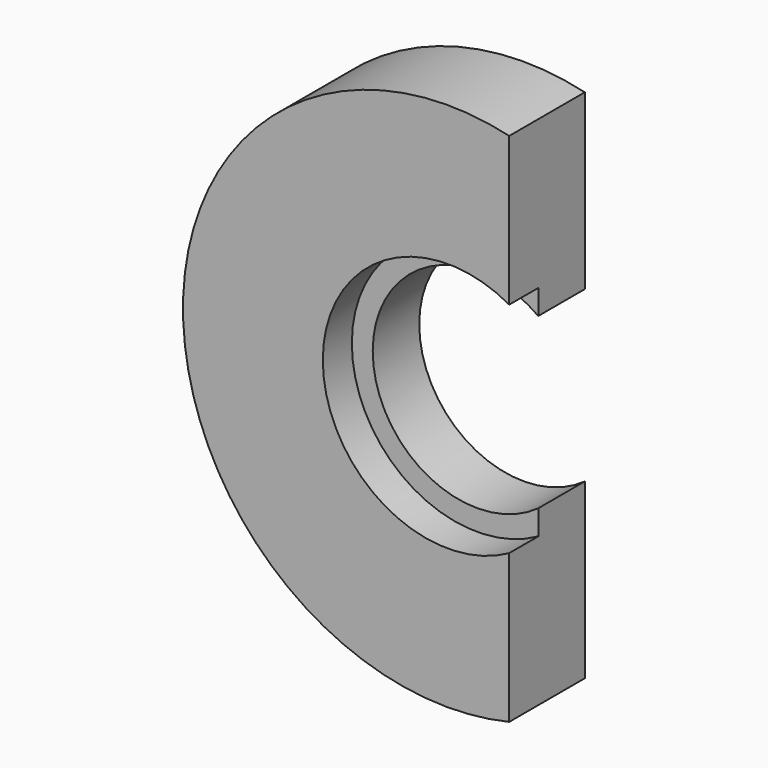
from build123d import *

# Parameters (mm, degrees)
F6_DEPTH = 9.501


# Not quite as in the source:
# - a feature of the source that left no trace in its solid (it failed there, or was rolled back) is left out
# - the program builds the solid bodies; features that only make, move or delete a surface that nothing else refers to are left out


with BuildPart() as f4:
    # F0 (on Top) → F4 (revolve)
    with BuildSketch(Plane.XY):
        Polygon((34.4624469289, 70.1398981537), (36.5624469289, 70.1398981537), (36.5624469289, 75.9898981537), (20.4008240253, 75.9898981537), (20.4008240253, 66.4898981537), (28.4008240253, 66.4898981537), (34.4624469289, 66.4898981537), align=None)
    revolve(axis=Axis((47.0624469289, 47.4898981537, 0), (0, -1, 0)))

    # F5 (on face) → F6 (cut, through all)
    with BuildSketch(Plane(origin=(0, 75.9898981537, 0), x_dir=(-1, 0, 0), z_dir=(0, 1, 0))):
        with BuildLine():
            Line((-53.2110722647, 8.511427993), (-53.2110722647, 25.9429478343))
            ThreePointArc((-53.2110722647, 25.9429478343), (-73.7240698325, 0), (-53.2110722647, -25.9429478343))
            Line((-53.2110722647, -25.9429478343), (-53.2110722647, -8.511427993))
            ThreePointArc((-53.2110722647, -8.511427993), (-57.5624469289, 0), (-53.2110722647, 8.511427993))
        make_face()
    extrude(amount=-F6_DEPTH, mode=Mode.SUBTRACT)


solid = f4.part
